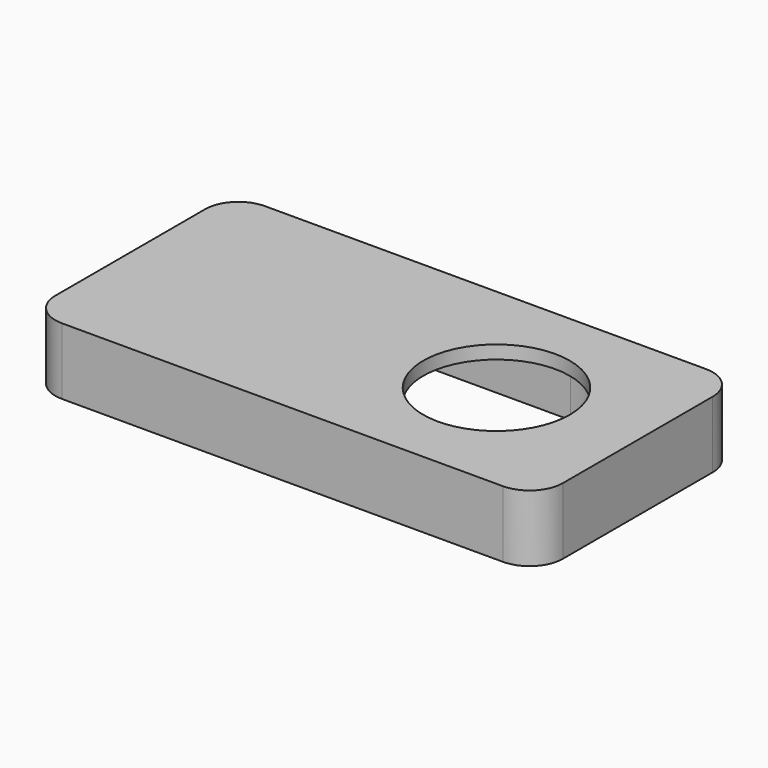
from build123d import *

# Parameters (mm, degrees)
F1_DEPTH = 10
F2_R     = 11
F3_DEPTH = 20
F5_DEPTH = 6
F7_DEPTH = 8


# Not quite as in the source:
# - a feature names something its author has since deleted; it is built from what else it names


with BuildPart() as f1:
    # F0 (on Top) → F1 (new body)
    with BuildSketch(Plane.XY):
        with BuildLine():
            Line((33.1, 19.05), (-33.1, 19.05))
            ThreePointArc((-33.1, 19.05), (-36.6355339059, 17.5855339059), (-38.1, 14.05))
            Line((-38.1, 14.05), (-38.1, -14.05))
            ThreePointArc((-38.1, -14.05), (-36.6355339059, -17.5855339059), (-33.1, -19.05))
            Line((-33.1, -19.05), (33.1, -19.05))
            ThreePointArc((33.1, -19.05), (36.6355339059, -17.5855339059), (38.1, -14.05))
            Line((38.1, -14.05), (38.1, 14.05))
            ThreePointArc((38.1, 14.05), (36.6355339059, 17.5855339059), (33.1, 19.05))
        make_face()
    extrude(amount=F1_DEPTH)

    # F2 (on Top) → F3 (cut)
    with BuildSketch(Plane.XY):
        with Locations((16.8899707496, 0)):
            Circle(F2_R)
    extrude(amount=F3_DEPTH, mode=Mode.SUBTRACT)

    # F4 (on Top) → F5 (cut)
    with BuildSketch(Plane.XY):
        with BuildLine():
            Line((31, -14), (31, -11.625))
            ThreePointArc((31, -11.625), (29.3206213947, -12.3206213947), (28.625, -14))
            Line((28.625, -14), (31, -14))
        make_face()
        with BuildLine():
            ThreePointArc((33.375, -14), (32.6793786053, -12.3206213947), (31, -11.625))
            Line((31, -11.625), (31, -14))
            Line((31, -14), (28.625, -14))
            ThreePointArc((28.625, -14), (31, -16.375), (33.375, -14))
        make_face()
        with BuildLine():
            ThreePointArc((-28.625, -14), (-29.3206213947, -12.3206213947), (-31, -11.625))
            Line((-31, -11.625), (-31, -14))
            Line((-31, -14), (-28.625, -14))
        make_face()
        with BuildLine():
            Line((-31, -14), (-31, -11.625))
            ThreePointArc((-31, -11.625), (-32.6793786053, -15.6793786053), (-28.625, -14))
            Line((-28.625, -14), (-31, -14))
        make_face()
        with BuildLine():
            Line((-31, 14), (-28.625, 14))
            ThreePointArc((-28.625, 14), (-32.6793786053, 15.6793786053), (-31, 11.625))
            Line((-31, 11.625), (-31, 14))
        make_face()
        with BuildLine():
            ThreePointArc((-31, 11.625), (-29.3206213947, 12.3206213947), (-28.625, 14))
            Line((-28.625, 14), (-31, 14))
            Line((-31, 14), (-31, 11.625))
        make_face()
        with BuildLine():
            Line((31, 14), (28.625, 14))
            ThreePointArc((28.625, 14), (29.3206213947, 12.3206213947), (31, 11.625))
            Line((31, 11.625), (31, 14))
        make_face()
        with BuildLine():
            ThreePointArc((33.375, 14), (31, 16.375), (28.625, 14))
            Line((28.625, 14), (31, 14))
            Line((31, 14), (31, 11.625))
            ThreePointArc((31, 11.625), (32.6793786053, 12.3206213947), (33.375, 14))
        make_face()
    extrude(amount=F5_DEPTH, mode=Mode.SUBTRACT)

    # F6 (on Top) → F7 (cut)
    with BuildSketch(Plane.XY):
        with BuildLine():
            Line((16.8287921697, 14), (-18, 14))
            ThreePointArc((-18, 14), (-27.8994949366, 9.8994949366), (-32, 0))
            ThreePointArc((-32, 0), (-27.8994949366, -9.8994949366), (-18, -14))
            Line((-18, -14), (16.8287921697, -14))
            ThreePointArc((16.8287921697, -14), (26.7282871063, -9.8994949366), (30.8287921697, 0))
            ThreePointArc((30.8287921697, 0), (26.7282871063, 9.8994949366), (16.8287921697, 14))
        make_face()
    extrude(amount=F7_DEPTH, mode=Mode.SUBTRACT)


solid = f1.part
